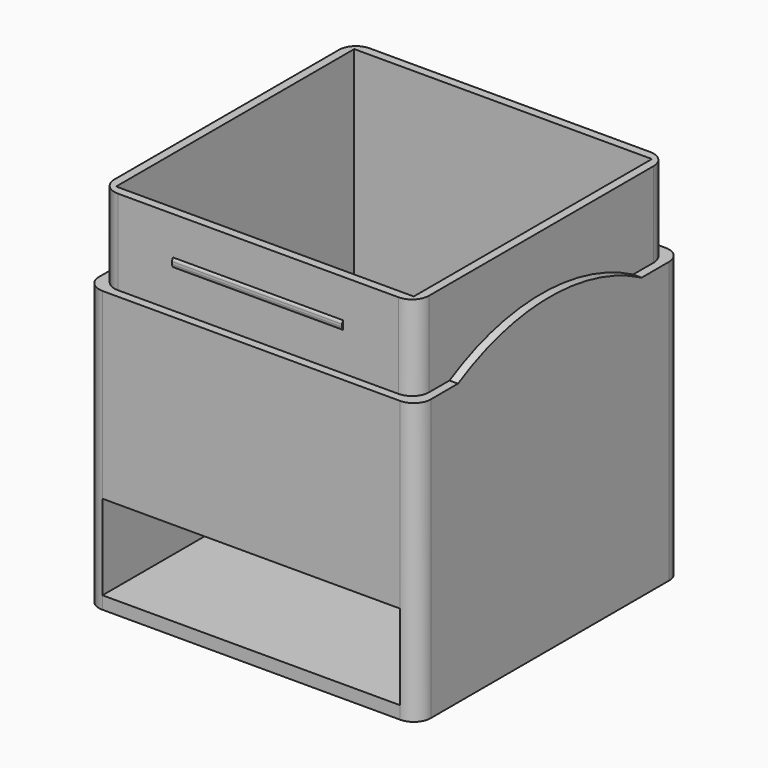
from build123d import *

# Parameters (mm, degrees)
F0_W         = 78
F0_H         = 78
F1_DEPTH     = 86
F2_T         = -4
F4_DEPTH     = 24
F3_W         = 70
F3_H         = 20
F5_DEPTH     = 74
F6_W         = 78
F6_H         = 78
F6_W_2       = 74
F6_H_2       = 74
F7_DEPTH     = 20
F9_DEPTH     = 2
F10_R        = 3.99999
F11_R        = 4
F12_W        = 40
F12_H        = 2
F13_DEPTH    = 0.3
F14_T1_DEPTH = 43.5707142143
F15_T1_DEPTH = 43.5707142143


# Not quite as in the source:
# - a fillet or chamfer that OpenCascade refuses, or shapes differently, is made with other operations: its cross-section is extruded or revolved along the edge and cut away or added
# - a fillet or chamfer is up to 0.001 mm smaller than in the source, because OpenCascade refuses the exact size


with BuildPart() as f1:
    # F0 (on Top) → F1 (new body)
    with BuildSketch(Plane.XY):
        with Locations((-38.7419309749, 20.0862393249)):
            Rectangle(F0_W, F0_H)
    extrude(amount=F1_DEPTH)

    # F2
    f2_openings = [f1.faces().sort_by_distance(p)[0] for p in [
        (-38.741931, 20.086239, 86),
    ]]
    offset(amount=F2_T, openings=f2_openings)

    # F4 (add): a face of the model
    f4_faces = [f1.faces().sort_by_distance(p)[0] for p in [
        (-38.7419309749, 20.0862393249, 4),
    ]]
    extrude(f4_faces, amount=F4_DEPTH)

    # F3 (on face) → F5 (cut)
    with BuildSketch(Plane.XZ.offset(18.9137606751)):
        with Locations((-38.7419309749, 13)):
            Rectangle(F3_W, F3_H)
    extrude(amount=-F5_DEPTH, mode=Mode.SUBTRACT)

    # F6 (on face) → F7 (cut)
    with BuildSketch(Plane.XY.offset(86)):
        with Locations((-38.7419309749, 20.0862393249)):
            Rectangle(F6_W, F6_H)
        with Locations((-38.7419309749, 20.0862393249)):
            Rectangle(F6_W_2, F6_H_2, mode=Mode.SUBTRACT)
    extrude(amount=-F7_DEPTH, mode=Mode.SUBTRACT)

    # F8 (on face) → F9 (join)
    with BuildSketch(Plane.YZ.offset(-1.7419309749)):
        with BuildLine():
            Line((-6.9137606751, 66), (47.0862393249, 66))
            ThreePointArc((47.0862393249, 66), (20.0862393249, 73), (-6.9137606751, 66))
        make_face()
    extrude(amount=F9_DEPTH)

    # F10 (radius 4 in the source; OpenCascade refuses exactly that, so slightly less here)
    f10_edges = [f1.edges().sort_by_distance(p)[0] for p in [
        (-77.741931, -18.913761, 33),
        (0.258069, -18.913761, 33),
        (0.258069, 59.086239, 33),
        (-77.741931, 59.086239, 33),
    ]]
    fillet(f10_edges, radius=F10_R)

    # F11
    f11_edges = [f1.edges().sort_by_distance(p)[0] for p in [
        (-1.741931, -16.913761, 76),
        (-1.741931, 57.086239, 76),
        (-75.741931, -16.913761, 76),
        (-75.741931, 57.086239, 76),
    ]]
    fillet(f11_edges, radius=F11_R)

    # F12 (on face) → F13 (join)
    with BuildSketch(Plane.XZ.offset(16.9137606751)):
        with Locations((-38.7419309749, 76)):
            Rectangle(F12_W, F12_H)
    extrude(amount=F13_DEPTH)

    # F14: fillet of radius 1 on 1 edges, made by hand

    # F14_s2 → F14_t1 (cut)
    with BuildSketch(Plane.YZ.offset(-60.527288082)):
        with BuildLine():
            ThreePointArc((-16.9137606751, 77), (-17.1357151208, 76.6731554918), (-17.2137606751, 76.2858571571))
            Line((-17.2137606751, 76.2858571571), (-17.2137606751, 77))
            Line((-17.2137606751, 77), (-16.9137606751, 77))
        make_face()
    extrude(amount=F14_T1_DEPTH, mode=Mode.SUBTRACT)

    # F15: fillet of radius 1 on 1 edges, made by hand

    # F15_s2 → F15_t1 (cut)
    with BuildSketch(Plane.YZ.offset(-60.527288082)):
        with BuildLine():
            ThreePointArc((-16.9137606751, 75), (-17.1357151208, 75.3268445082), (-17.2137606751, 75.7141428429))
            Line((-17.2137606751, 75.7141428429), (-17.2137606751, 75))
            Line((-17.2137606751, 75), (-16.9137606751, 75))
        make_face()
    extrude(amount=F15_T1_DEPTH, mode=Mode.SUBTRACT)


solid = f1.part
